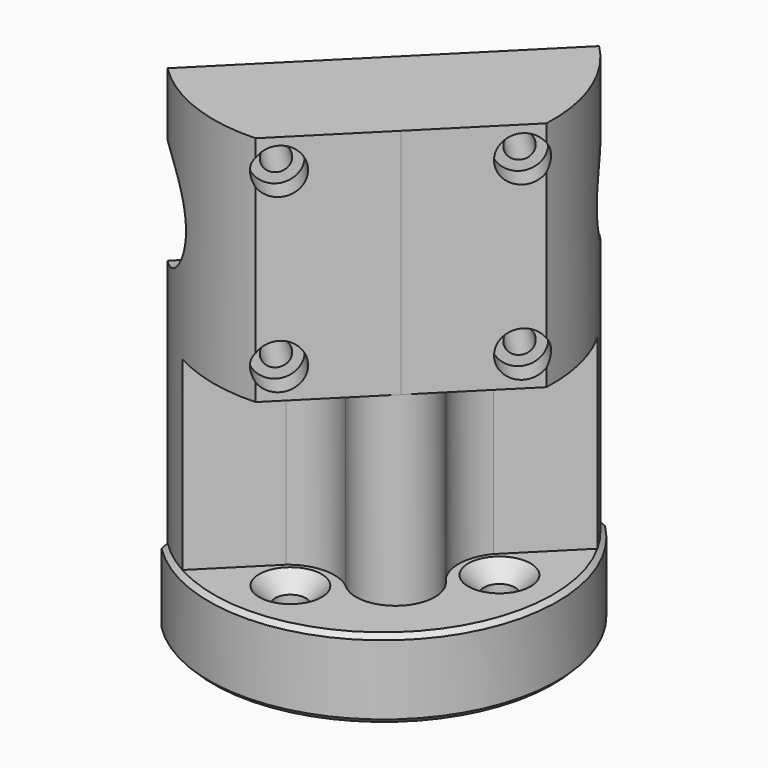
from build123d import *

# Parameters (mm, degrees)
F1_ANGLE_BACK   = 45
F1_ANGLE        = 180
F2_SIZE         = 1
F4_D            = 6.6
F4_CSINK_D      = 13.44
F4_CSINK_ANGLE  = 90
F6_DEPTH        = 40
F8_DEPTH        = 50
F12_D           = 5.5
F12_CBORE_D     = 9.75
F12_CBORE_DEPTH = 5


# Not quite as in the source:
# - a feature names something its author has since deleted; it is built from what else it names


with BuildPart() as f1:
    # F0 (on Front) → F1 (revolve)
    with BuildSketch(Plane.XZ, mode=Mode.PRIVATE) as f1_sk:
        Polygon((0, 10), (0, 0), (31.6, 0), (31.6, -7), (37.5, -7), (37.5, 10), align=None)
    revolve(f1_sk.sketch.rotate(Axis((0, 0, 5), (0, 0, -1)), -F1_ANGLE_BACK), axis=Axis((0, 0, 5), (0, 0, -1)), revolution_arc=F1_ANGLE)

    # F2
    f2_edges = [f1.edges().sort_by_distance(p)[0] for p in [
        (22.344574, -22.344574, -7),
        (26.516504, -26.516504, -7),
        (26.516504, -26.516504, 10),
    ]]
    chamfer(f2_edges, length=F2_SIZE)

    # F4 (through all)
    with Locations(Plane.XY.offset(10)):
        with Locations((25, 0), (0, -25)):
            CounterSinkHole(F4_D / 2, F4_CSINK_D / 2, counter_sink_angle=F4_CSINK_ANGLE)

    # F5 (on face) → F6 (join)
    with BuildSketch(Plane.XY.offset(10)):
        with BuildLine():
            Line((19.4820004924, 5.3398648686), (7.0710678119, -7.0710678119))
            Line((7.0710678119, -7.0710678119), (-5.3398648686, -19.4820004924))
            ThreePointArc((-5.3398648686, -19.4820004924), (0.79408889, -17.1167209324), (7.0710678119, -19.0710678119))
            ThreePointArc((7.0710678119, -19.0710678119), (19.0710678119, -19.0710678119), (19.0710678119, -7.0710678119))
            ThreePointArc((19.0710678119, -7.0710678119), (17.1167209324, -0.79408889), (19.4820004924, 5.3398648686))
        make_face()
        with BuildLine():
            Line((7.0710678119, -7.0710678119), (0, 0))
            Line((0, 0), (-25.8093975133, -25.8093975133))
            ThreePointArc((-25.8093975133, -25.8093975133), (-21.9914756212, -29.1311688746), (-17.7507975491, -31.8929331729))
            Line((-17.7507975491, -31.8929331729), (-5.3398648686, -19.4820004924))
            Line((-5.3398648686, -19.4820004924), (7.0710678119, -7.0710678119))
        make_face()
        with BuildLine():
            Line((25.8093975133, 25.8093975133), (0, 0))
            Line((0, 0), (7.0710678119, -7.0710678119))
            Line((7.0710678119, -7.0710678119), (19.4820004924, 5.3398648686))
            Line((19.4820004924, 5.3398648686), (31.8929331729, 17.7507975491))
            ThreePointArc((31.8929331729, 17.7507975491), (29.1311688746, 21.9914756212), (25.8093975133, 25.8093975133))
        make_face()
    extrude(amount=F6_DEPTH)

    # F7 (on face) → F8 (join)
    with BuildSketch(Plane.XY.offset(50)):
        with BuildLine():
            ThreePointArc((36.4612769111, -1.6808587126), (35.531279534, 8.3533331479), (31.8929331729, 17.7507975491))
            Line((31.8929331729, 17.7507975491), (19.4820004924, 5.3398648686))
            ThreePointArc((19.4820004924, 5.3398648686), (17.1167209324, -0.79408889), (19.0710678119, -7.0710678119))
            ThreePointArc((19.0710678119, -7.0710678119), (21.5563491861, -13.0710678119), (19.0710678119, -19.0710678119))
            Line((19.0710678119, -19.0710678119), (36.4612769111, -1.6808587126))
        make_face()
        with BuildLine():
            Line((-5.3398648686, -19.4820004924), (-17.7507975491, -31.8929331729))
            ThreePointArc((-17.7507975491, -31.8929331729), (-8.3533331479, -35.531279534), (1.6808587126, -36.4612769111))
            Line((1.6808587126, -36.4612769111), (19.0710678119, -19.0710678119))
            ThreePointArc((19.0710678119, -19.0710678119), (13.0710678119, -21.5563491861), (7.0710678119, -19.0710678119))
            ThreePointArc((7.0710678119, -19.0710678119), (0.79408889, -17.1167209324), (-5.3398648686, -19.4820004924))
        make_face()
        with BuildLine():
            ThreePointArc((31.8929331729, 17.7507975491), (29.1311688746, 21.9914756212), (25.8093975133, 25.8093975133))
            Line((25.8093975133, 25.8093975133), (-25.8093975133, -25.8093975133))
            ThreePointArc((-25.8093975133, -25.8093975133), (-21.9914756212, -29.1311688746), (-17.7507975491, -31.8929331729))
            Line((-17.7507975491, -31.8929331729), (-5.3398648686, -19.4820004924))
            ThreePointArc((-5.3398648686, -19.4820004924), (0.79408889, -17.1167209324), (7.0710678119, -19.0710678119))
            ThreePointArc((7.0710678119, -19.0710678119), (13.0710678119, -21.5563491861), (19.0710678119, -19.0710678119))
            ThreePointArc((19.0710678119, -19.0710678119), (21.5563491861, -13.0710678119), (19.0710678119, -7.0710678119))
            ThreePointArc((19.0710678119, -7.0710678119), (17.1167209324, -0.79408889), (19.4820004924, 5.3398648686))
            Line((19.4820004924, 5.3398648686), (31.8929331729, 17.7507975491))
        make_face()
    extrude(amount=F8_DEPTH)

    # F9 (on face) → F10 (revolve, cut)
    with BuildSketch(Plane(origin=(0, 0, 0), x_dir=(-0.7071067812, -0.7071067812, 0), z_dir=(-0.7071067812, 0.7071067812, 0))):
        Polygon((36.5, 86.5), (-36.5, 85.5), (-36.5, 75), (36.5, 75), align=None)
    revolve(axis=Axis((0, 0, 75), (-0.7071067812, -0.7071067812, 0)), mode=Mode.SUBTRACT)

    # F12 (through all)
    with Locations(Plane(origin=(19.0710678119, -19.0710678119, 0), x_dir=(0.7071067812, 0.7071067812, 0), z_dir=(0.7071067812, -0.7071067812, 0))):
        with Locations((20.5934695606, 93.5), (20.5934695606, 56.5), (-20.5934695606, 56.5), (-20.5934695606, 93.5)):
            CounterBoreHole(F12_D / 2, F12_CBORE_D / 2, F12_CBORE_DEPTH)


solid = f1.part
